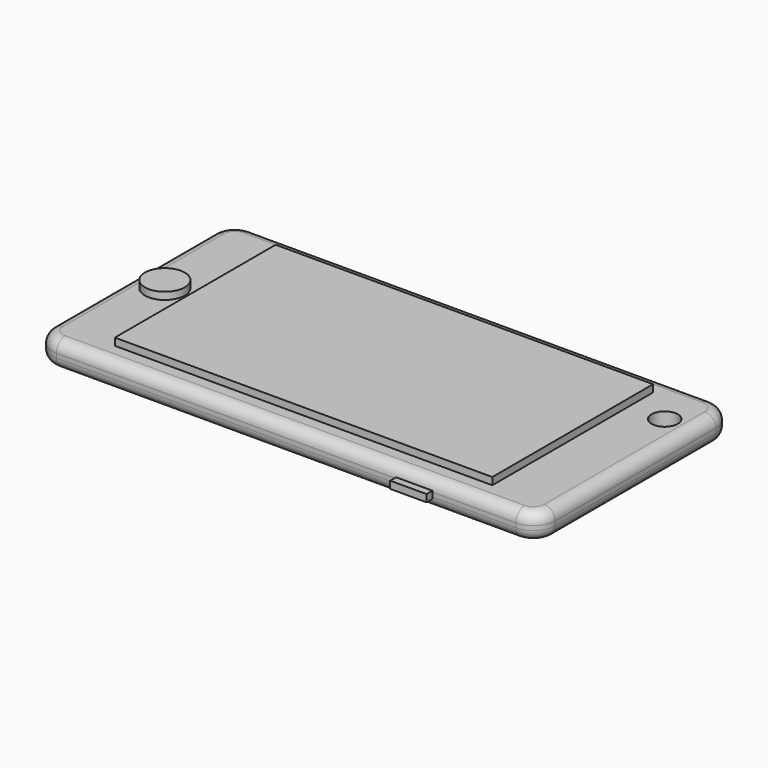
from build123d import *

# Parameters (mm, degrees)
F0_R          = 3.6
F1_DEPTH      = 7.2
F2_W          = 5.5
F2_H          = 2.4
F3_DEPTH      = 1
F4_W          = 10
F4_H          = 2
F5_DEPTH      = 2
F6_W          = 8.8
F6_H          = 3
F7_DEPTH      = 5
F8_R          = 5.5
F9_DEPTH      = 2
F10_W         = 103.9
F10_H         = 55.33
F11_DEPTH     = 2
F12_T1_DEPTH  = 55.3
F12_T6_DEPTH  = 126.45
F12_T12_DEPTH = 126.45
F12_T18_DEPTH = 126.45
F12_T25_DEPTH = 126.45
F12_T31_DEPTH = 126.45
F12_T35_ANGLE = 90
F12_T39_DEPTH = 126.45
F12_T45_DEPTH = 126.45
F12_T51_DEPTH = 126.45
F12_T58_DEPTH = 126.45
F12_T64_DEPTH = 126.45
F12_T68_ANGLE = 90
F12_T70_ANGLE = 90
F12_T72_ANGLE = 90
F13_T1_DEPTH  = 55.3
F13_T6_DEPTH  = 126.45
F13_T12_DEPTH = 126.45
F13_T18_DEPTH = 126.45
F13_T25_DEPTH = 126.45
F13_T31_DEPTH = 126.45
F13_T35_ANGLE = 90
F13_T37_ANGLE = 90
F13_T41_DEPTH = 126.45
F13_T47_DEPTH = 126.45
F13_T53_DEPTH = 126.45
F13_T60_DEPTH = 126.45
F13_T66_DEPTH = 126.45
F13_T70_ANGLE = 90
F13_T72_ANGLE = 90


# Not quite as in the source:
# - a fillet or chamfer that OpenCascade refuses, or shapes differently, is made with other operations: its cross-section is extruded or revolved along the edge and cut away or added


with BuildPart() as f1:
    # F0 (on Top) → F1 (new body)
    with BuildSketch(Plane.XY):
        with BuildLine():
            Line((63.225, 33.65), (-63.225, 33.65))
            ThreePointArc((-63.225, 33.65), (-67.4676406871, 31.8926406871), (-69.225, 27.65))
            Line((-69.225, 27.65), (-69.225, -27.65))
            ThreePointArc((-69.225, -27.65), (-67.4676406871, -31.8926406871), (-63.225, -33.65))
            Line((-63.225, -33.65), (63.225, -33.65))
            ThreePointArc((63.225, -33.65), (67.4676406871, -31.8926406871), (69.225, -27.65))
            Line((69.225, -27.65), (69.225, 27.65))
            ThreePointArc((69.225, 27.65), (67.4676406871, 31.8926406871), (63.225, 33.65))
        make_face()
        with Locations((61.625, 19.55)):
            Circle(F0_R, mode=Mode.SUBTRACT)
    extrude(amount=F1_DEPTH)

    # F2 (on face) → F3 (join)
    with BuildSketch(Plane(origin=(0, 33.65, 0), x_dir=(-1, 0, 0), z_dir=(0, 1, 0))):
        with Locations((-48.275, 3.7285785931)):
            Rectangle(F2_W, F2_H)
    extrude(amount=F3_DEPTH)

    # F4 (on face) → F5 (join)
    with BuildSketch(Plane.XZ.offset(33.65)):
        with Locations((35.225, 3.5)):
            Rectangle(F4_W, F4_H)
    extrude(amount=F5_DEPTH)

    # F6 (on face) → F7 (cut)
    with BuildSketch(Plane(origin=(-69.225, 0, 0), x_dir=(0, -1, 0), z_dir=(-1, 0, 0))):
        with Locations((0, 3.3)):
            Rectangle(F6_W, F6_H)
    extrude(amount=-F7_DEPTH, mode=Mode.SUBTRACT)

    # F8 (on face) → F9 (join)
    with BuildSketch(Plane.XY.offset(7.2)):
        with Locations((-60.325, 0)):
            Circle(F8_R)
    extrude(amount=F9_DEPTH)

    # F10 (on face) → F11 (join)
    with BuildSketch(Plane.XY.offset(7.2)):
        Rectangle(F10_W, F10_H)
    extrude(amount=F11_DEPTH)

    # F12: fillet of radius 3 on 8 edges, made by hand

    # F12_s2 → F12_t1 (cut)
    with BuildSketch(Plane.XZ.offset(-27.65)):
        with BuildLine():
            ThreePointArc((-66.225, 7.2), (-68.3463203436, 6.3213203436), (-69.225, 4.2))
            Line((-69.225, 4.2), (-69.225, 7.2))
            Line((-69.225, 7.2), (-66.225, 7.2))
        make_face()
        with BuildLine():
            ThreePointArc((66.225, 7.2), (68.3463203436, 6.3213203436), (69.225, 4.2))
            Line((69.225, 4.2), (69.225, 7.2))
            Line((69.225, 7.2), (66.225, 7.2))
        make_face()
    extrude(amount=F12_T1_DEPTH, mode=Mode.SUBTRACT)


with BuildPart() as f12_tool4:
    # F12_s5 → F12_t6 (new body)
    with BuildSketch(Plane.YZ.offset(63.225)):
        with BuildLine():
            ThreePointArc((33.65, 4.2), (32.7713203436, 6.3213203436), (30.65, 7.2))
            Line((30.65, 7.2), (33.65, 7.2))
            Line((33.65, 7.2), (33.65, 4.2))
        make_face()
    extrude(amount=-F12_T6_DEPTH)

    split(bisect_by=Plane.XY.offset(4.9285785931), keep=Keep.BOTTOM)

    split(bisect_by=Plane.YZ.offset(51.025), keep=Keep.TOP)


with BuildPart() as f1_1:
    add(f1.part)

    # F12_t3: cut F12_tool4
    add(f12_tool4.part, mode=Mode.SUBTRACT)


with BuildPart() as f12_tool10:
    # F12_s11 → F12_t12 (new body)
    with BuildSketch(Plane.YZ.offset(63.225)):
        with BuildLine():
            ThreePointArc((33.65, 4.2), (32.7713203436, 6.3213203436), (30.65, 7.2))
            Line((30.65, 7.2), (33.65, 7.2))
            Line((33.65, 7.2), (33.65, 4.2))
        make_face()
    extrude(amount=-F12_T12_DEPTH)

    split(bisect_by=Plane.XY.offset(4.9285785931), keep=Keep.TOP)

    split(bisect_by=Plane.YZ.offset(51.025), keep=Keep.TOP)


with BuildPart() as f1_2:
    add(f1_1.part)

    # F12_t9: cut F12_tool10
    add(f12_tool10.part, mode=Mode.SUBTRACT)


with BuildPart() as f12_tool16:
    # F12_s17 → F12_t18 (new body)
    with BuildSketch(Plane.YZ.offset(63.225)):
        with BuildLine():
            ThreePointArc((33.65, 4.2), (32.7713203436, 6.3213203436), (30.65, 7.2))
            Line((30.65, 7.2), (33.65, 7.2))
            Line((33.65, 7.2), (33.65, 4.2))
        make_face()
    extrude(amount=-F12_T18_DEPTH)

    split(bisect_by=Plane.XY.offset(4.9285785931), keep=Keep.TOP)

    split(bisect_by=Plane.YZ.offset(45.525), keep=Keep.TOP)

    split(bisect_by=Plane.YZ.offset(51.025), keep=Keep.BOTTOM)


with BuildPart() as f1_3:
    add(f1_2.part)

    # F12_t15: cut F12_tool16
    add(f12_tool16.part, mode=Mode.SUBTRACT)


with BuildPart() as f12_tool23:
    # F12_s24 → F12_t25 (new body)
    with BuildSketch(Plane.YZ.offset(63.225)):
        with BuildLine():
            ThreePointArc((33.65, 4.2), (32.7713203436, 6.3213203436), (30.65, 7.2))
            Line((30.65, 7.2), (33.65, 7.2))
            Line((33.65, 7.2), (33.65, 4.2))
        make_face()
    extrude(amount=-F12_T25_DEPTH)

    split(bisect_by=Plane.XY.offset(4.9285785931), keep=Keep.BOTTOM)

    split(bisect_by=Plane.YZ.offset(45.525), keep=Keep.BOTTOM)


with BuildPart() as f1_4:
    add(f1_3.part)

    # F12_t22: cut F12_tool23
    add(f12_tool23.part, mode=Mode.SUBTRACT)


with BuildPart() as f12_tool29:
    # F12_s30 → F12_t31 (new body)
    with BuildSketch(Plane.YZ.offset(63.225)):
        with BuildLine():
            ThreePointArc((33.65, 4.2), (32.7713203436, 6.3213203436), (30.65, 7.2))
            Line((30.65, 7.2), (33.65, 7.2))
            Line((33.65, 7.2), (33.65, 4.2))
        make_face()
    extrude(amount=-F12_T31_DEPTH)

    split(bisect_by=Plane.XY.offset(4.9285785931), keep=Keep.TOP)

    split(bisect_by=Plane.YZ.offset(45.525), keep=Keep.BOTTOM)


with BuildPart() as f1_5:
    add(f1_4.part)

    # F12_t28: cut F12_tool29
    add(f12_tool29.part, mode=Mode.SUBTRACT)

    # F12_s34 → F12_t35 (revolve, cut)
    with BuildSketch(Plane.YZ.offset(-63.225)):
        with BuildLine():
            ThreePointArc((30.65, 7.2), (32.7713203436, 6.3213203436), (33.65, 4.2))
            Line((33.65, 4.2), (33.65, 7.2))
            Line((33.65, 7.2), (30.65, 7.2))
        make_face()
    revolve(axis=Axis((-63.225, 27.65, 7.2), (0, 0, 1)), revolution_arc=F12_T35_ANGLE, mode=Mode.SUBTRACT)


with BuildPart() as f12_tool37:
    # F12_s38 → F12_t39 (new body)
    with BuildSketch(Plane.YZ.offset(-63.225)):
        with BuildLine():
            ThreePointArc((-30.65, 7.2), (-32.7713203436, 6.3213203436), (-33.65, 4.2))
            Line((-33.65, 4.2), (-33.65, 7.2))
            Line((-33.65, 7.2), (-30.65, 7.2))
        make_face()
    extrude(amount=F12_T39_DEPTH)

    split(bisect_by=Plane.YZ.offset(30.225), keep=Keep.BOTTOM)

    split(bisect_by=Plane.XY.offset(4.5), keep=Keep.TOP)


with BuildPart() as f1_6:
    add(f1_5.part)

    # F12_t36: cut F12_tool37
    add(f12_tool37.part, mode=Mode.SUBTRACT)


with BuildPart() as f12_tool43:
    # F12_s44 → F12_t45 (new body)
    with BuildSketch(Plane.YZ.offset(-63.225)):
        with BuildLine():
            ThreePointArc((-30.65, 7.2), (-32.7713203436, 6.3213203436), (-33.65, 4.2))
            Line((-33.65, 4.2), (-33.65, 7.2))
            Line((-33.65, 7.2), (-30.65, 7.2))
        make_face()
    extrude(amount=F12_T45_DEPTH)

    split(bisect_by=Plane.YZ.offset(30.225), keep=Keep.BOTTOM)

    split(bisect_by=Plane.XY.offset(4.5), keep=Keep.BOTTOM)


with BuildPart() as f1_7:
    add(f1_6.part)

    # F12_t42: cut F12_tool43
    add(f12_tool43.part, mode=Mode.SUBTRACT)


with BuildPart() as f12_tool49:
    # F12_s50 → F12_t51 (new body)
    with BuildSketch(Plane.YZ.offset(-63.225)):
        with BuildLine():
            ThreePointArc((-30.65, 7.2), (-32.7713203436, 6.3213203436), (-33.65, 4.2))
            Line((-33.65, 4.2), (-33.65, 7.2))
            Line((-33.65, 7.2), (-30.65, 7.2))
        make_face()
    extrude(amount=F12_T51_DEPTH)

    split(bisect_by=Plane.YZ.offset(30.225), keep=Keep.TOP)

    split(bisect_by=Plane.XY.offset(4.5), keep=Keep.TOP)

    split(bisect_by=Plane.YZ.offset(40.225), keep=Keep.BOTTOM)


with BuildPart() as f1_8:
    add(f1_7.part)

    # F12_t48: cut F12_tool49
    add(f12_tool49.part, mode=Mode.SUBTRACT)


with BuildPart() as f12_tool56:
    # F12_s57 → F12_t58 (new body)
    with BuildSketch(Plane.YZ.offset(-63.225)):
        with BuildLine():
            ThreePointArc((-30.65, 7.2), (-32.7713203436, 6.3213203436), (-33.65, 4.2))
            Line((-33.65, 4.2), (-33.65, 7.2))
            Line((-33.65, 7.2), (-30.65, 7.2))
        make_face()
    extrude(amount=F12_T58_DEPTH)

    split(bisect_by=Plane.XY.offset(4.5), keep=Keep.TOP)

    split(bisect_by=Plane.YZ.offset(40.225), keep=Keep.TOP)


with BuildPart() as f1_9:
    add(f1_8.part)

    # F12_t55: cut F12_tool56
    add(f12_tool56.part, mode=Mode.SUBTRACT)


with BuildPart() as f12_tool62:
    # F12_s63 → F12_t64 (new body)
    with BuildSketch(Plane.YZ.offset(-63.225)):
        with BuildLine():
            ThreePointArc((-30.65, 7.2), (-32.7713203436, 6.3213203436), (-33.65, 4.2))
            Line((-33.65, 4.2), (-33.65, 7.2))
            Line((-33.65, 7.2), (-30.65, 7.2))
        make_face()
    extrude(amount=F12_T64_DEPTH)

    split(bisect_by=Plane.XY.offset(4.5), keep=Keep.BOTTOM)

    split(bisect_by=Plane.YZ.offset(40.225), keep=Keep.TOP)


with BuildPart() as f1_10:
    add(f1_9.part)

    # F12_t61: cut F12_tool62
    add(f12_tool62.part, mode=Mode.SUBTRACT)

    # F12_s67 → F12_t68 (revolve, cut)
    with BuildSketch(Plane.XZ.offset(27.65)):
        with BuildLine():
            ThreePointArc((-66.225, 7.2), (-68.3463203436, 6.3213203436), (-69.225, 4.2))
            Line((-69.225, 4.2), (-69.225, 7.2))
            Line((-69.225, 7.2), (-66.225, 7.2))
        make_face()
    revolve(axis=Axis((-63.225, -27.65, 7.2), (0, 0, 1)), revolution_arc=F12_T68_ANGLE, mode=Mode.SUBTRACT)

    # F12_s69 → F12_t70 (revolve, cut)
    with BuildSketch(Plane.YZ.offset(63.225)):
        with BuildLine():
            ThreePointArc((-30.65, 7.2), (-32.7713203436, 6.3213203436), (-33.65, 4.2))
            Line((-33.65, 4.2), (-33.65, 7.2))
            Line((-33.65, 7.2), (-30.65, 7.2))
        make_face()
    revolve(axis=Axis((63.225, -27.65, 7.2), (0, 0, 1)), revolution_arc=F12_T70_ANGLE, mode=Mode.SUBTRACT)

    # F12_s71 → F12_t72 (revolve, cut)
    with BuildSketch(Plane.XZ.offset(-27.65)):
        with BuildLine():
            ThreePointArc((69.225, 4.2), (68.3463203436, 6.3213203436), (66.225, 7.2))
            Line((66.225, 7.2), (69.225, 7.2))
            Line((69.225, 7.2), (69.225, 4.2))
        make_face()
    revolve(axis=Axis((63.225, 27.65, 7.2), (0, 0, 1)), revolution_arc=F12_T72_ANGLE, mode=Mode.SUBTRACT)

    # F13: fillet of radius 3 on 8 edges, made by hand

    # F13_s2 → F13_t1 (cut)
    with BuildSketch(Plane.XZ.offset(-27.65)):
        with BuildLine():
            ThreePointArc((-66.225, 0), (-68.3463203436, 0.8786796564), (-69.225, 3))
            Line((-69.225, 3), (-69.225, 0))
            Line((-69.225, 0), (-66.225, 0))
        make_face()
        with BuildLine():
            ThreePointArc((66.225, 0), (68.3463203436, 0.8786796564), (69.225, 3))
            Line((69.225, 3), (69.225, 0))
            Line((69.225, 0), (66.225, 0))
        make_face()
    extrude(amount=F13_T1_DEPTH, mode=Mode.SUBTRACT)


with BuildPart() as f13_tool4:
    # F13_s5 → F13_t6 (new body)
    with BuildSketch(Plane.YZ.offset(-63.225)):
        with BuildLine():
            ThreePointArc((-30.65, 0), (-32.7713203436, 0.8786796564), (-33.65, 3))
            Line((-33.65, 3), (-33.65, 0))
            Line((-33.65, 0), (-30.65, 0))
        make_face()
    extrude(amount=F13_T6_DEPTH)

    split(bisect_by=Plane.XY.offset(2.5), keep=Keep.BOTTOM)

    split(bisect_by=Plane.YZ.offset(30.225), keep=Keep.BOTTOM)


with BuildPart() as f1_11:
    add(f1_10.part)

    # F13_t3: cut F13_tool4
    add(f13_tool4.part, mode=Mode.SUBTRACT)


with BuildPart() as f13_tool10:
    # F13_s11 → F13_t12 (new body)
    with BuildSketch(Plane.YZ.offset(-63.225)):
        with BuildLine():
            ThreePointArc((-30.65, 0), (-32.7713203436, 0.8786796564), (-33.65, 3))
            Line((-33.65, 3), (-33.65, 0))
            Line((-33.65, 0), (-30.65, 0))
        make_face()
    extrude(amount=F13_T12_DEPTH)

    split(bisect_by=Plane.XY.offset(2.5), keep=Keep.TOP)

    split(bisect_by=Plane.YZ.offset(30.225), keep=Keep.BOTTOM)


with BuildPart() as f1_12:
    add(f1_11.part)

    # F13_t9: cut F13_tool10
    add(f13_tool10.part, mode=Mode.SUBTRACT)


with BuildPart() as f13_tool16:
    # F13_s17 → F13_t18 (new body)
    with BuildSketch(Plane.YZ.offset(-63.225)):
        with BuildLine():
            ThreePointArc((-30.65, 0), (-32.7713203436, 0.8786796564), (-33.65, 3))
            Line((-33.65, 3), (-33.65, 0))
            Line((-33.65, 0), (-30.65, 0))
        make_face()
    extrude(amount=F13_T18_DEPTH)

    split(bisect_by=Plane.YZ.offset(40.225), keep=Keep.BOTTOM)

    split(bisect_by=Plane.XY.offset(2.5), keep=Keep.BOTTOM)

    split(bisect_by=Plane.YZ.offset(30.225), keep=Keep.TOP)


with BuildPart() as f1_13:
    add(f1_12.part)

    # F13_t15: cut F13_tool16
    add(f13_tool16.part, mode=Mode.SUBTRACT)


with BuildPart() as f13_tool23:
    # F13_s24 → F13_t25 (new body)
    with BuildSketch(Plane.YZ.offset(-63.225)):
        with BuildLine():
            ThreePointArc((-30.65, 0), (-32.7713203436, 0.8786796564), (-33.65, 3))
            Line((-33.65, 3), (-33.65, 0))
            Line((-33.65, 0), (-30.65, 0))
        make_face()
    extrude(amount=F13_T25_DEPTH)

    split(bisect_by=Plane.YZ.offset(40.225), keep=Keep.TOP)

    split(bisect_by=Plane.XY.offset(2.5), keep=Keep.BOTTOM)


with BuildPart() as f1_14:
    add(f1_13.part)

    # F13_t22: cut F13_tool23
    add(f13_tool23.part, mode=Mode.SUBTRACT)


with BuildPart() as f13_tool29:
    # F13_s30 → F13_t31 (new body)
    with BuildSketch(Plane.YZ.offset(-63.225)):
        with BuildLine():
            ThreePointArc((-30.65, 0), (-32.7713203436, 0.8786796564), (-33.65, 3))
            Line((-33.65, 3), (-33.65, 0))
            Line((-33.65, 0), (-30.65, 0))
        make_face()
    extrude(amount=F13_T31_DEPTH)

    split(bisect_by=Plane.YZ.offset(40.225), keep=Keep.TOP)

    split(bisect_by=Plane.XY.offset(2.5), keep=Keep.TOP)


with BuildPart() as f1_15:
    add(f1_14.part)

    # F13_t28: cut F13_tool29
    add(f13_tool29.part, mode=Mode.SUBTRACT)

    # F13_s34 → F13_t35 (revolve, cut)
    with BuildSketch(Plane.XZ.offset(27.65)):
        with BuildLine():
            ThreePointArc((-66.225, 0), (-68.3463203436, 0.8786796564), (-69.225, 3))
            Line((-69.225, 3), (-69.225, 0))
            Line((-69.225, 0), (-66.225, 0))
        make_face()
    revolve(axis=Axis((-63.225, -27.65, 0), (0, 0, 1)), revolution_arc=F13_T35_ANGLE, mode=Mode.SUBTRACT)

    # F13_s36 → F13_t37 (revolve, cut)
    with BuildSketch(Plane.YZ.offset(-63.225)):
        with BuildLine():
            ThreePointArc((30.65, 0), (32.7713203436, 0.8786796564), (33.65, 3))
            Line((33.65, 3), (33.65, 0))
            Line((33.65, 0), (30.65, 0))
        make_face()
    revolve(axis=Axis((-63.225, 27.65, 0), (0, 0, 1)), revolution_arc=F13_T37_ANGLE, mode=Mode.SUBTRACT)


with BuildPart() as f13_tool39:
    # F13_s40 → F13_t41 (new body)
    with BuildSketch(Plane.YZ.offset(63.225)):
        with BuildLine():
            ThreePointArc((33.65, 3), (32.7713203436, 0.8786796564), (30.65, 0))
            Line((30.65, 0), (33.65, 0))
            Line((33.65, 0), (33.65, 3))
        make_face()
    extrude(amount=-F13_T41_DEPTH)

    split(bisect_by=Plane.XY.offset(2.5285785931), keep=Keep.TOP)

    split(bisect_by=Plane.YZ.offset(51.025), keep=Keep.TOP)


with BuildPart() as f1_16:
    add(f1_15.part)

    # F13_t38: cut F13_tool39
    add(f13_tool39.part, mode=Mode.SUBTRACT)


with BuildPart() as f13_tool45:
    # F13_s46 → F13_t47 (new body)
    with BuildSketch(Plane.YZ.offset(63.225)):
        with BuildLine():
            ThreePointArc((33.65, 3), (32.7713203436, 0.8786796564), (30.65, 0))
            Line((30.65, 0), (33.65, 0))
            Line((33.65, 0), (33.65, 3))
        make_face()
    extrude(amount=-F13_T47_DEPTH)

    split(bisect_by=Plane.XY.offset(2.5285785931), keep=Keep.BOTTOM)

    split(bisect_by=Plane.YZ.offset(51.025), keep=Keep.TOP)


with BuildPart() as f1_17:
    add(f1_16.part)

    # F13_t44: cut F13_tool45
    add(f13_tool45.part, mode=Mode.SUBTRACT)


with BuildPart() as f13_tool51:
    # F13_s52 → F13_t53 (new body)
    with BuildSketch(Plane.YZ.offset(63.225)):
        with BuildLine():
            ThreePointArc((33.65, 3), (32.7713203436, 0.8786796564), (30.65, 0))
            Line((30.65, 0), (33.65, 0))
            Line((33.65, 0), (33.65, 3))
        make_face()
    extrude(amount=-F13_T53_DEPTH)

    split(bisect_by=Plane.YZ.offset(45.525), keep=Keep.TOP)

    split(bisect_by=Plane.XY.offset(2.5285785931), keep=Keep.BOTTOM)

    split(bisect_by=Plane.YZ.offset(51.025), keep=Keep.BOTTOM)


with BuildPart() as f1_18:
    add(f1_17.part)

    # F13_t50: cut F13_tool51
    add(f13_tool51.part, mode=Mode.SUBTRACT)


with BuildPart() as f13_tool58:
    # F13_s59 → F13_t60 (new body)
    with BuildSketch(Plane.YZ.offset(63.225)):
        with BuildLine():
            ThreePointArc((33.65, 3), (32.7713203436, 0.8786796564), (30.65, 0))
            Line((30.65, 0), (33.65, 0))
            Line((33.65, 0), (33.65, 3))
        make_face()
    extrude(amount=-F13_T60_DEPTH)

    split(bisect_by=Plane.YZ.offset(45.525), keep=Keep.BOTTOM)

    split(bisect_by=Plane.XY.offset(2.5285785931), keep=Keep.TOP)


with BuildPart() as f1_19:
    add(f1_18.part)

    # F13_t57: cut F13_tool58
    add(f13_tool58.part, mode=Mode.SUBTRACT)


with BuildPart() as f13_tool64:
    # F13_s65 → F13_t66 (new body)
    with BuildSketch(Plane.YZ.offset(63.225)):
        with BuildLine():
            ThreePointArc((33.65, 3), (32.7713203436, 0.8786796564), (30.65, 0))
            Line((30.65, 0), (33.65, 0))
            Line((33.65, 0), (33.65, 3))
        make_face()
    extrude(amount=-F13_T66_DEPTH)

    split(bisect_by=Plane.YZ.offset(45.525), keep=Keep.BOTTOM)

    split(bisect_by=Plane.XY.offset(2.5285785931), keep=Keep.BOTTOM)


with BuildPart() as f1_20:
    add(f1_19.part)

    # F13_t63: cut F13_tool64
    add(f13_tool64.part, mode=Mode.SUBTRACT)

    # F13_s69 → F13_t70 (revolve, cut)
    with BuildSketch(Plane.XZ.offset(-27.65)):
        with BuildLine():
            ThreePointArc((66.225, 0), (68.3463203436, 0.8786796564), (69.225, 3))
            Line((69.225, 3), (69.225, 0))
            Line((69.225, 0), (66.225, 0))
        make_face()
    revolve(axis=Axis((63.225, 27.65, 0), (0, 0, 1)), revolution_arc=F13_T70_ANGLE, mode=Mode.SUBTRACT)

    # F13_s71 → F13_t72 (revolve, cut)
    with BuildSketch(Plane.YZ.offset(63.225)):
        with BuildLine():
            ThreePointArc((-30.65, 0), (-32.7713203436, 0.8786796564), (-33.65, 3))
            Line((-33.65, 3), (-33.65, 0))
            Line((-33.65, 0), (-30.65, 0))
        make_face()
    revolve(axis=Axis((63.225, -27.65, 0), (0, 0, 1)), revolution_arc=F13_T72_ANGLE, mode=Mode.SUBTRACT)


solid = f1_20.part
